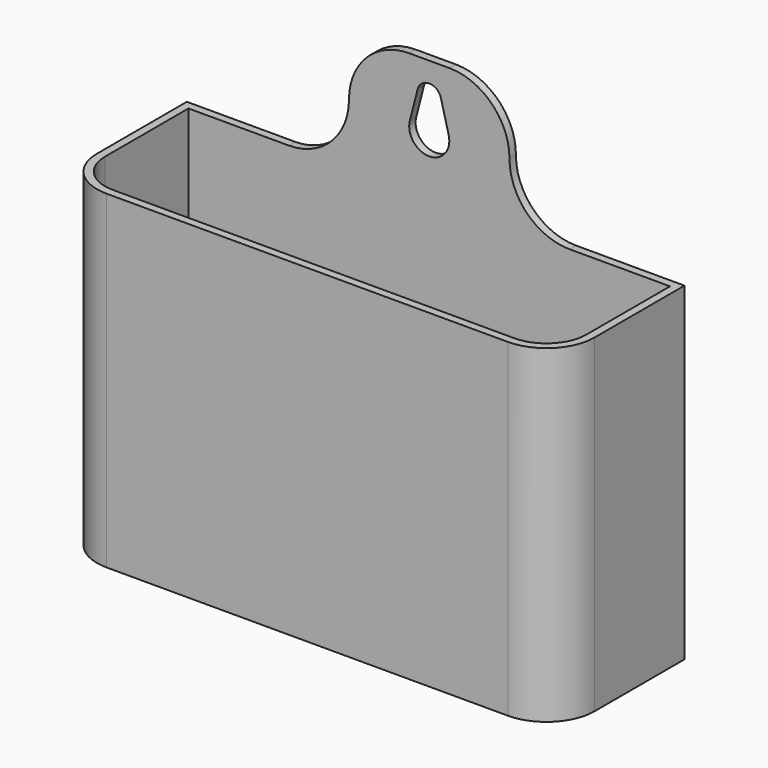
from build123d import *

# Parameters (mm, degrees)
F0_W     = 62
F0_H     = 20
F1_DEPTH = 1
F2_W     = 62
F2_H     = 20
F2_W_2   = 60
F2_H_2   = 18
F3_DEPTH = 40
F4_R     = 5
F5_R     = 6
F6_W     = 20
F6_H     = 1
F7_DEPTH = 15
F9_DEPTH = 1
F10_R    = 7.49999


# Not quite as in the source:
# - a fillet or chamfer is up to 0.001 mm smaller than in the source, because OpenCascade refuses the exact size


with BuildPart() as f1:
    # F0 (on Top) → F1 (new body)
    with BuildSketch(Plane.XY):
        with Locations((31, 10)):
            Rectangle(F0_W, F0_H)
    extrude(amount=F1_DEPTH)

    # F2 (on face) → F3 (join)
    with BuildSketch(Plane.XY.offset(1)):
        with Locations((31, 10)):
            Rectangle(F2_W, F2_H)
        with Locations((31, 10)):
            Rectangle(F2_W_2, F2_H_2, mode=Mode.SUBTRACT)
    extrude(amount=F3_DEPTH)

    # F4
    f4_edges = [f1.edges().sort_by_distance(p)[0] for p in [
        (1, 1, 21),
        (61, 1, 21),
    ]]
    fillet(f4_edges, radius=F4_R)

    # F5
    f5_edges = [f1.edges().sort_by_distance(p)[0] for p in [
        (0, 0, 20.5),
        (62, 0, 20.5),
    ]]
    fillet(f5_edges, radius=F5_R)

    # F6 (on face) → F7 (join)
    with BuildSketch(Plane.XY.offset(41)):
        with Locations((31, 19.5)):
            Rectangle(F6_W, F6_H)
    extrude(amount=F7_DEPTH)

    # F8 (on face) → F9 (cut, through all)
    with BuildSketch(Plane.XZ.offset(-19)):
        with BuildLine():
            Line((33.4206145914, 48.625), (32.4523687548, 52.375))
            ThreePointArc((32.4523687548, 52.375), (31, 53.5), (29.5476312452, 52.375))
            Line((29.5476312452, 52.375), (28.5793854086, 48.625))
            ThreePointArc((28.5793854086, 48.625), (31, 45.5), (33.4206145914, 48.625))
        make_face()
    extrude(amount=-F9_DEPTH, mode=Mode.SUBTRACT)

    # F10 (radius 7.5 in the source; OpenCascade refuses exactly that, so slightly less here)
    f10_edges = [f1.edges().sort_by_distance(p)[0] for p in [
        (21, 19.5, 56),
        (41, 19.5, 56),
        (41, 19.5, 41),
        (21, 19.5, 41),
    ]]
    fillet(f10_edges, radius=F10_R)


solid = f1.part
